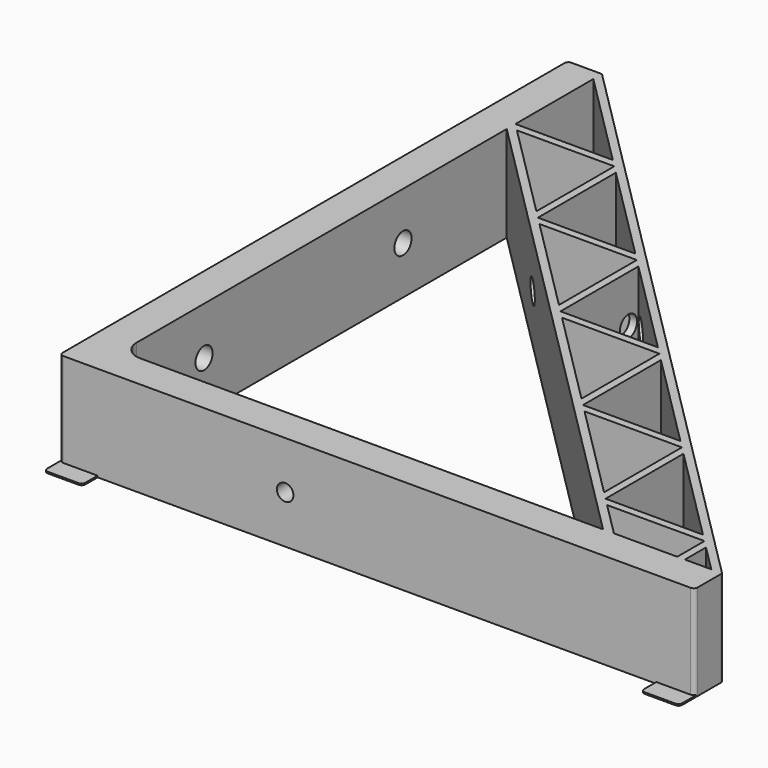
from build123d import *

# Parameters (mm, degrees)
F0_W           = 2
F0_H           = 9
F1_DEPTH       = 25
F3_D           = 5.6134
F3_DEPTH       = 25
F3_TIP         = 1.6864354994
F5_D           = 5.6134
F5_DEPTH       = 85
F5_TIP         = 1.6864354994
F7_D           = 4.318
F7_DEPTH       = 25
F7_CSINK_D     = 7.7978
F7_CSINK_ANGLE = 82
F7_TIP         = 1.2972580765
F8_R           = 5
F9_R           = 1
F11_DEPTH      = 0.4
F12_R          = 1


# Not quite as in the source:
# - a feature names something its author has since deleted; it is built from what else it names


with BuildPart() as f1:
    # F0 (on Top) → F1 (new body)
    with BuildSketch(Plane.XY):
        Polygon((0, 166), (0, 0), (154.2796328583, 0), (154.2796328583, 9), (137.7157287525, 9), (134.8873016278, 9), (9, 9), (9, 134.8873016278), (9, 137.7157287525), (9, 138.1715728753), (9, 163.1715728753), (9, 166), align=None)
        Polygon((36.4558441227, 135.7157287525), (34.4558441227, 137.7157287525), (9, 137.7157287525), (11, 135.7157287525), align=None)
        Polygon((38.4558441227, 133.7157287525), (36.4558441227, 135.7157287525), (36.4558441227, 110.2598846298), (38.4558441227, 108.2598846298), align=None)
        Polygon((134.8873016278, 9), (137.7157287525, 9), (128.8237887356, 17.891940017), (126.8237887356, 19.891940017), (126.8236856744, 19.8920430782), (124.8236856744, 21.8920430782), (99.3678415517, 47.3478872009), (97.3678415517, 49.3478872009), (97.3677384905, 49.347990262), (95.3677384905, 51.347990262), (69.9118943678, 76.8038343848), (67.9118943678, 78.8038343848), (67.9117913066, 78.8039374459), (65.9117913066, 80.8039374459), (40.4559471839, 106.2597815687), (38.4559471839, 108.2597815687), (38.4558441227, 108.2598846298), (36.4558441227, 110.2598846298), (11, 135.7157287525), (9, 137.7157287525), (9, 134.8873016278), align=None)
        Polygon((166, 9), (9, 166), (9, 163.1715728753), (34.4558441227, 137.7157287525), (36.4558441227, 135.7157287525), (38.4558441227, 133.7157287525), (63.9117913066, 108.2597815687), (65.9117913066, 106.2597815687), (67.9117913066, 104.2597815687), (93.3677384905, 78.8038343848), (95.3677384905, 76.8038343848), (97.3677384905, 74.8038343848), (122.8236856744, 49.3478872009), (124.8236856744, 47.3478872009), (126.8236856744, 45.3478872009), (150.2702352589, 21.9013376164), (152.2796328583, 19.891940017), (154.2796328583, 17.891940017), (156.2796328583, 15.891940017), (163.1715728753, 9), align=None)
        Polygon((65.9117913066, 106.2597815687), (63.9117913066, 108.2597815687), (38.4559471839, 108.2597815687), (40.4559471839, 106.2597815687), align=None)
        Polygon((67.9117913066, 104.2597815687), (65.9117913066, 106.2597815687), (65.9117913066, 80.8039374459), (67.9117913066, 78.8039374459), align=None)
        Polygon((95.3677384905, 76.8038343848), (93.3677384905, 78.8038343848), (67.9118943678, 78.8038343848), (69.9118943678, 76.8038343848), align=None)
        Polygon((97.3677384905, 49.347990262), (97.3677384905, 74.8038343848), (95.3677384905, 76.8038343848), (95.3677384905, 51.347990262), align=None)
        Polygon((99.3678415517, 47.3478872009), (124.8236856744, 47.3478872009), (122.8236856744, 49.3478872009), (97.3678415517, 49.3478872009), align=None)
        Polygon((124.8236856744, 21.8920430782), (126.8236856744, 19.8920430782), (126.8236856744, 45.3478872009), (124.8236856744, 47.3478872009), align=None)
        Polygon((128.8237887356, 17.891940017), (154.2796328583, 17.891940017), (152.2796328583, 19.891940017), (126.8237887356, 19.891940017), align=None)
        Polygon((154.2796328583, 17.891940017), (154.2796328583, 9), (156.2796328583, 9), (156.2796328583, 15.891940017), align=None)
        with Locations((155.2796328583, 4.5)):
            Rectangle(F0_W, F0_H)
        Polygon((156.2796328583, 9), (156.2796328583, 0), (166, 0), (166, 6.1715728753), (163.1715728753, 9), align=None)
        Polygon((166, 6.1715728753), (166, 9), (163.1715728753, 9), align=None)
    extrude(amount=F1_DEPTH)

    # F3
    with Locations(Plane(origin=(0, 0, 0), x_dir=(0, -1, 0), z_dir=(-1, 0, 0))):
        with Locations((-36, 12.5)):
            Hole(F3_D / 2, depth=F3_DEPTH)
            with Locations((0, 0, -(F3_DEPTH + F3_TIP / 2))):  # 118° drill point
                Cone(0, F3_D / 2, F3_TIP, mode=Mode.SUBTRACT)

    # F5
    with Locations(Plane(origin=(0, 0, 0), x_dir=(0, -1, 0), z_dir=(-1, 0, 0))):
        with Locations((-101, 12.5)):
            Hole(F5_D / 2, depth=F5_DEPTH)
            with Locations((0, 0, -(F5_DEPTH + F5_TIP / 2))):  # 118° drill point
                Cone(0, F5_D / 2, F5_TIP, mode=Mode.SUBTRACT)

    # F7
    with Locations(Plane(origin=(0, 9, 0), x_dir=(-1, 0, 0), z_dir=(0, 1, 0))):
        with Locations((-59, 12.5)):
            CounterSinkHole(F7_D / 2, F7_CSINK_D / 2, depth=F7_DEPTH, counter_sink_angle=F7_CSINK_ANGLE)
            with Locations((0, 0, -(F7_DEPTH + F7_TIP / 2))):  # 118° drill point
                Cone(0, F7_D / 2, F7_TIP, mode=Mode.SUBTRACT)

    # F8
    f8_edges = [f1.edges().sort_by_distance(p)[0] for p in [
        (9, 9, 12.5),
    ]]
    fillet(f8_edges, radius=F8_R)

    # F9
    f9_edges = [f1.edges().sort_by_distance(p)[0] for p in [
        (166, 9, 12.5),
        (166, 0, 12.5),
        (0, 0, 12.5),
        (0, 166, 12.5),
        (9, 166, 12.5),
    ]]
    fillet(f9_edges, radius=F9_R)

    # F10 (on face) → F11 (join)
    with BuildSketch(Plane(origin=(0, 0, 0), x_dir=(1, 0, 0), z_dir=(0, 0, -1))):
        with BuildLine():
            Line((156, 5), (156, 0))
            Line((156, 0), (165, 0))
            ThreePointArc((165, 0), (165.5171897304, -0.1441292254), (165.8852951503, -0.5349704344))
            Line((165.8852951503, -0.5349704344), (166, -0.5349704344))
            Line((166, -0.5349704344), (166, 5))
            Line((166, 5), (156, 5))
        make_face()
        with BuildLine():
            Line((0, 5), (0, -1))
            ThreePointArc((0, -1), (0.2928932188, -0.2928932188), (1, 0))
            Line((1, 0), (10, 0))
            Line((10, 0), (10, 5))
            Line((10, 5), (0, 5))
        make_face()
    extrude(amount=-F11_DEPTH)

    # F12
    f12_edges = [f1.edges().sort_by_distance(p)[0] for p in [
        (166, -5, 0.2),
        (156, -5, 0.2),
        (0, -5, 0.2),
        (10, -5, 0.2),
    ]]
    fillet(f12_edges, radius=F12_R)


solid = f1.part
